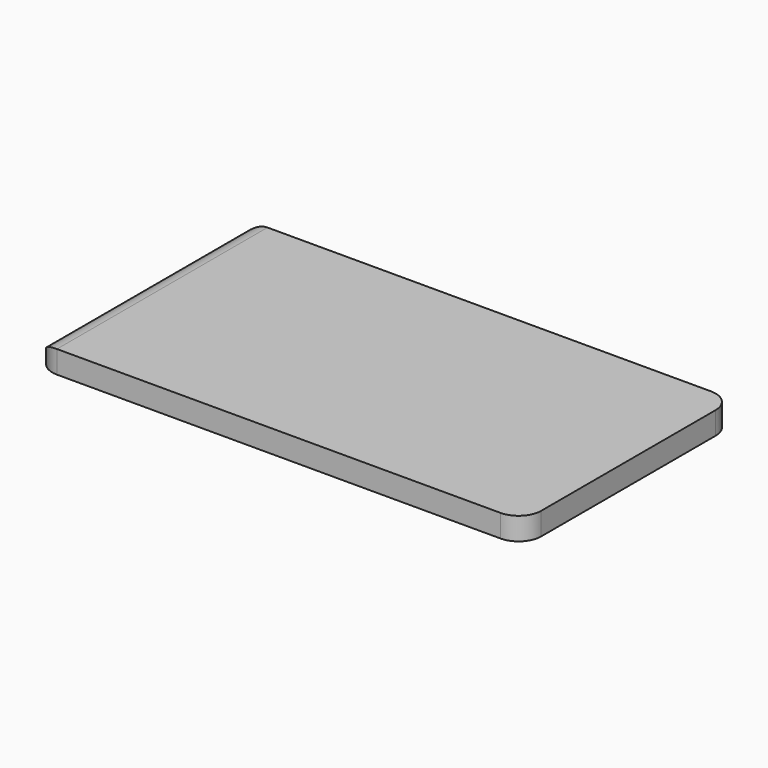
from build123d import *

# Parameters (mm, degrees)
F0_W        = 65
F0_H        = 35
F1_DEPTH    = 3
F2_R        = 3
F3_T1_DEPTH = 44


# Not quite as in the source:
# - a fillet or chamfer that OpenCascade refuses, or shapes differently, is made with other operations: its cross-section is extruded or revolved along the edge and cut away or added


with BuildPart() as f1:
    # F0 (on Top) → F1 (new body)
    with BuildSketch(Plane.XY):
        Rectangle(F0_W, F0_H)
    extrude(amount=-F1_DEPTH)

    # F2
    f2_edges = [f1.edges().sort_by_distance(p)[0] for p in [
        (-32.5, -17.5, -1.5),
        (-32.5, 17.5, -1.5),
        (32.5, 17.5, -1.5),
        (32.5, -17.5, -1.5),
    ]]
    fillet(f2_edges, radius=F2_R)

    # F3: fillet of radius 3 on 1 edges, made by hand

    # F3_s2 → F3_t1 (cut)
    with BuildSketch(Plane.XZ.offset(-22)):
        with BuildLine():
            ThreePointArc((-29.5, 0), (-31.6213203436, -0.8786796564), (-32.5, -3))
            Line((-32.5, -3), (-32.5, 0))
            Line((-32.5, 0), (-29.5, 0))
        make_face()
    extrude(amount=F3_T1_DEPTH, mode=Mode.SUBTRACT)


solid = f1.part
